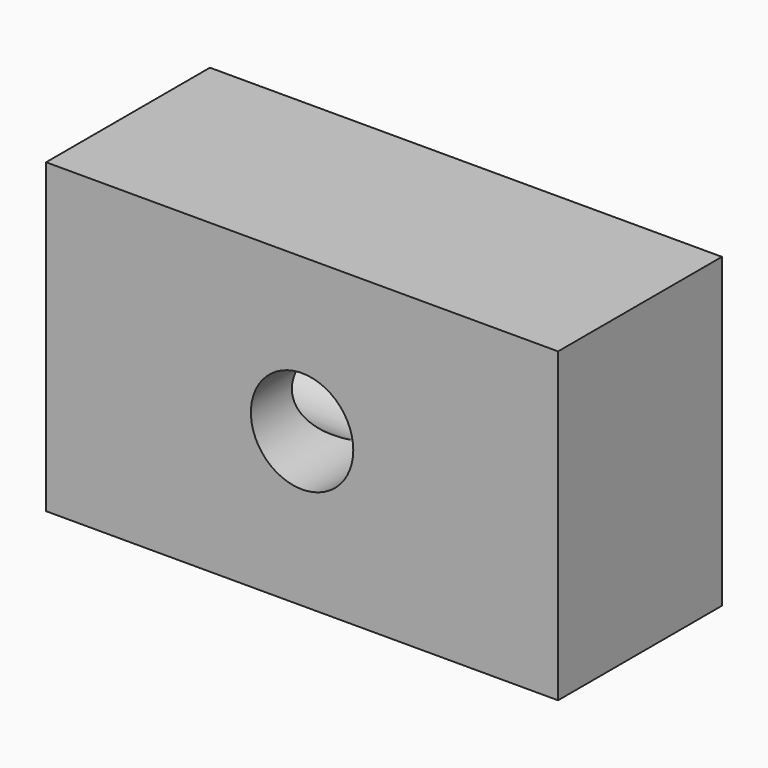
from build123d import *

# Parameters (mm, degrees)
F0_W     = 127
F0_H     = 76.2
F1_DEPTH = 50.8
F2_R     = 12.7
F3_DEPTH = 38.1
F4_R     = 12.7
F5_DEPTH = 76.2


# Not quite as in the source:
# - a feature of the source that left no trace in its solid (it failed there, or was rolled back) is left out


with BuildPart() as f1:
    # F0 (on Front) → F1 (new body)
    with BuildSketch(Plane.XZ):
        with Locations((31.5876135826, 9.5468121529)):
            Rectangle(F0_W, F0_H)
    extrude(amount=F1_DEPTH)

    # F2 (on face) → F3 (cut)
    with BuildSketch(Plane.XZ.offset(50.8)):
        with Locations((31.5876135826, 9.5468121529)):
            Circle(F2_R)
    extrude(amount=-F3_DEPTH, mode=Mode.SUBTRACT)

    # F4 (on face) → F5 (cut)
    with BuildSketch(Plane(origin=(-31.9123864174, 0, 0), x_dir=(0, -1, 0), z_dir=(-1, 0, 0))):
        with Locations((25.4, 9.5468121529)):
            Circle(F4_R)
    extrude(amount=-F5_DEPTH, mode=Mode.SUBTRACT)


solid = f1.part
